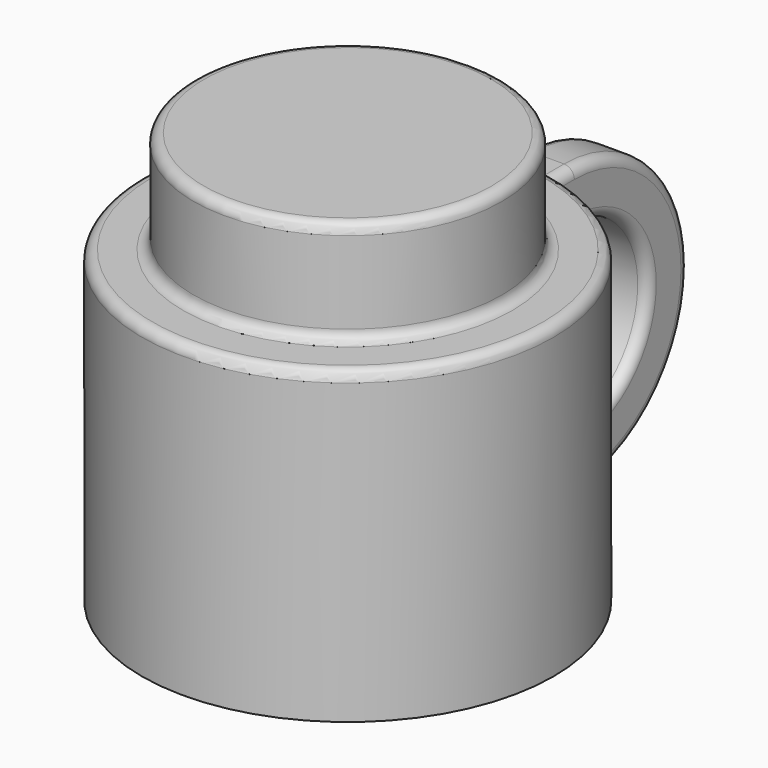
from build123d import *

# Parameters (mm, degrees)
F0_R          = 15
F1_DEPTH      = 10
F2_R          = 20
F3_DEPTH      = 30
F5_DEPTH      = 2.5
F5_DEPTH_BACK = 2.5
F7_DEPTH      = 25
F8_W          = 23
F8_H          = 23
F9_DEPTH      = 25
F10_R         = 1


with BuildPart() as f1:
    # F0 (on Top) → F1 (new body)
    with BuildSketch(Plane.XY):
        Circle(F0_R)
    extrude(amount=F1_DEPTH)

    # F2 (on Top) → F3 (join)
    with BuildSketch(Plane.XY):
        Circle(F2_R)
    extrude(amount=-F3_DEPTH)

    # F4 (on Right) → F5 (join, two sides)
    with BuildSketch(Plane.YZ) as f5_sk:
        with BuildLine():
            ThreePointArc((24.3955058538, -30), (34.2598373067, -25.9140601285), (38.3457771782, -16.0497286756))
            ThreePointArc((38.3457771782, -16.0497286756), (34.2598373067, -6.1853972226), (24.3955058538, -2.0994573511))
            Line((24.3955058538, -2.0994573511), (17.0112717897, -7.5845918618))
            Line((17.0112717897, -7.5845918618), (15.4388935224, -5.3544416027))
            ThreePointArc((15.4388935224, -5.3544416027), (10.5016803992, -17.3033969985), (17.4980895184, -28.1755572213))
            Line((17.4980895184, -28.1755572213), (18.3211155236, -26.8716588616))
            Line((18.3211155236, -26.8716588616), (24.3955058538, -30))
        make_face()
        with BuildLine():
            Line((17.0112717897, -7.5845918618), (24.3955058538, -2.0994573511))
            ThreePointArc((24.3955058538, -2.0994573511), (19.6306389371, -2.9384315127), (15.4388935224, -5.3544416027))
            Line((15.4388935224, -5.3544416027), (17.0112717897, -7.5845918618))
        make_face()
        with BuildLine():
            ThreePointArc((15.4388935224, -5.3544416027), (19.6306389371, -2.9384315127), (24.3955058538, -2.0994573511))
            Line((24.3955058538, -2.0994573511), (13.1439510733, -2.0994573511))
            Line((13.1439510733, -2.0994573511), (15.4388935224, -5.3544416027))
        make_face()
        with BuildLine():
            Line((16.3464937359, -30), (24.3955058538, -30))
            ThreePointArc((24.3955058538, -30), (20.8281909127, -29.5361786954), (17.4980895184, -28.1755572213))
            Line((17.4980895184, -28.1755572213), (16.3464937359, -30))
        make_face()
        with BuildLine():
            ThreePointArc((17.4980895184, -28.1755572213), (20.8281909127, -29.5361786954), (24.3955058538, -30))
            Line((24.3955058538, -30), (18.3211155236, -26.8716588616))
            Line((18.3211155236, -26.8716588616), (17.4980895184, -28.1755572213))
        make_face()
    extrude(amount=F5_DEPTH)
    extrude(f5_sk.sketch, amount=-F5_DEPTH_BACK)

    # F6 (on face) → F7 (cut)
    with BuildSketch(Plane(origin=(-2.5, 0, 0), x_dir=(0, -1, 0), z_dir=(-1, 0, 0))):
        with BuildLine():
            Line((-19.843134833, -23.4803773318), (-19.843134833, -8.6190800193))
            ThreePointArc((-19.843134833, -8.6190800193), (-33.3457771782, -16.0497286756), (-19.843134833, -23.4803773318))
        make_face()
    extrude(amount=-F7_DEPTH, mode=Mode.SUBTRACT)

    # F8 (on face) → F9 (cut)
    with BuildSketch(Plane(origin=(0, 0, -30), x_dir=(1, 0, 0), z_dir=(0, 0, -1))):
        Rectangle(F8_W, F8_H)
    extrude(amount=-F9_DEPTH, mode=Mode.SUBTRACT)

    # F10
    f10_edges = [f1.edges().sort_by_distance(p)[0] for p in [
        (-15, 0, 10),
        (-20, 0, 0),
        (2.5, 22.11932, -2.099457),
        (-2.5, 38.345777, -16.049729),
        (2.5, 33.345777, -16.049729),
        (-15, 0, 0),
    ]]
    fillet(f10_edges, radius=F10_R)


solid = f1.part
